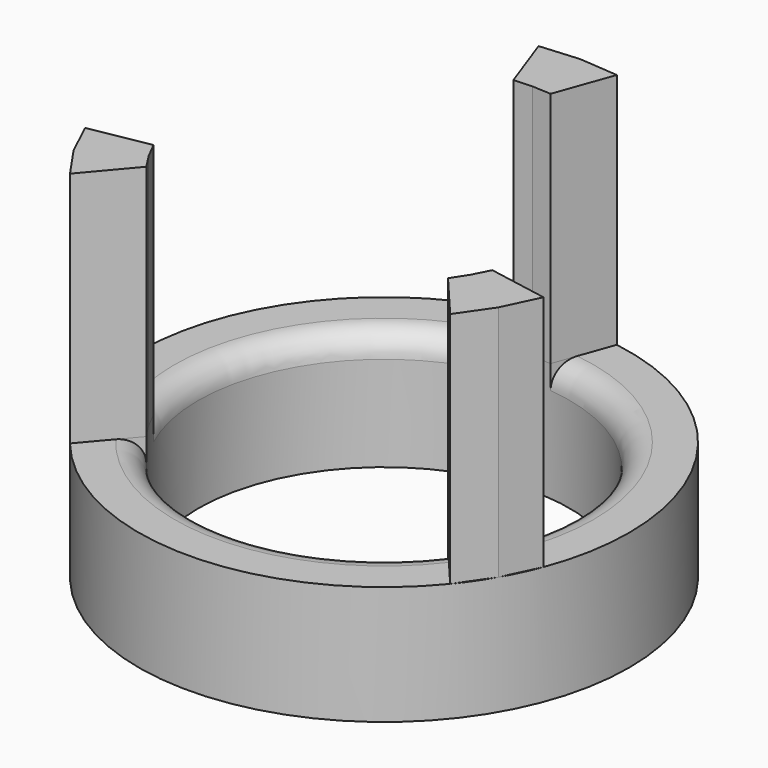
from build123d import *

# Parameters (mm, degrees)
F0_R         = 52.451
F0_R_2       = 39.751
F1_DEPTH     = 25.4
F3_DEPTH     = 50.8
F4_T4_ANGLE  = 145.1483416982
F4_T9_ANGLE  = 145.1483416982
F4_T16_ANGLE = 145.1483416982
F4_T23_ANGLE = 145.1483416982
F4_T28_ANGLE = 42.5640131775
F4_T33_ANGLE = 42.5640131775
F4_T38_ANGLE = 102.5699239424
F4_T44_ANGLE = 102.5699239424
F4_T49_ANGLE = 102.5699239424
F4_T54_ANGLE = 145.1483416982
F4_T59_ANGLE = 145.1483416982
F4_T66_ANGLE = 145.1483416982
F4_T73_ANGLE = 145.1483416982


# Not quite as in the source:
# - a fillet or chamfer that OpenCascade refuses, or shapes differently, is made with other operations: its cross-section is extruded or revolved along the edge and cut away or added


with BuildPart() as f1:
    # F0 (on Top) → F1 (new body)
    with BuildSketch(Plane.XY):
        Circle(F0_R)
        Circle(F0_R_2, mode=Mode.SUBTRACT)
    extrude(amount=F1_DEPTH)

    # F2 (on face) → F3 (join)
    with BuildSketch(Plane.XY.offset(25.4)):
        Polygon((0, 39.751), (3.9769716214, 39.5515574627), (8.3683463891, 51.7791288041), (0, 52.451), (-8.3683463891, 51.7791288041), (-3.9769716214, 39.5515574627), align=None)
        Polygon((-49.0262141247, -18.6423638414), (-45.4238984539, -26.2255), (-40.6578677356, -33.1367649627), (-32.2641677112, -23.2199371856), (-34.4253758258, -19.8755), (-36.2411393326, -16.331620277), align=None)
        Polygon((40.6578677356, -33.1367649627), (45.4238984539, -26.2255), (49.0262141247, -18.6423638414), (36.2411393326, -16.331620277), (34.4253758258, -19.8755), (32.2641677112, -23.2199371856), align=None)
    extrude(amount=F3_DEPTH)

    # F4: fillet of radius 5.08 on 4 edges, made by hand


with BuildPart() as f4_tool2:
    # F4_s3 → F4_t4 (revolve)
    with BuildSketch(Plane(origin=(0, 0, 0), x_dir=(0, 0, 1), z_dir=(0.9760150026, -0.2177032723, 0))):
        with BuildLine():
            ThreePointArc((25.4, -44.831), (23.9121024484, -41.2388975516), (20.32, -39.751))
            Line((20.32, -39.751), (25.4, -39.751))
            Line((25.4, -39.751), (25.4, -44.831))
        make_face()
    revolve(axis=Axis((0, 0, 25.4), (0, 0, 1)), revolution_arc=F4_T4_ANGLE)

    split(bisect_by=Plane(origin=(-9.0590317285, 3.2534345735, 0), x_dir=(0, 0, 1), z_dir=(0.9411459494, -0.3380004466, 0)), keep=Keep.TOP)


with BuildPart() as f1_1:
    add(f1.part)

    # F4_t1: cut F4_tool2
    add(f4_tool2.part, mode=Mode.SUBTRACT)


with BuildPart() as f4_tool7:
    # F4_s8 → F4_t9 (revolve)
    with BuildSketch(Plane(origin=(0, 0, 0), x_dir=(0, 0, 1), z_dir=(0.9760150026, -0.2177032723, 0))):
        with BuildLine():
            ThreePointArc((25.4, -44.831), (23.9121024484, -41.2388975516), (20.32, -39.751))
            Line((20.32, -39.751), (25.4, -39.751))
            Line((25.4, -39.751), (25.4, -44.831))
        make_face()
    revolve(axis=Axis((0, 0, 25.4), (0, 0, 1)), revolution_arc=F4_T9_ANGLE)

    split(bisect_by=Plane(origin=(9.0590317285, 3.2534345735, 0), x_dir=(0, 0, 1), z_dir=(-0.9411459494, -0.3380004466, 0)), keep=Keep.TOP)

    split(bisect_by=Plane(origin=(-33.3447717685, -21.5477185928, 0), x_dir=(0, 0, 1), z_dir=(0.8398952423, 0.542748544, 0)), keep=Keep.TOP)

    split(bisect_by=Plane(origin=(-35.3332575792, -18.1035601385, 0), x_dir=(0, 0, 1), z_dir=(0.8899816481, 0.4559963443, 0)), keep=Keep.TOP)


with BuildPart() as f1_2:
    add(f1_1.part)

    # F4_t6: cut F4_tool7
    add(f4_tool7.part, mode=Mode.SUBTRACT)


with BuildPart() as f4_tool14:
    # F4_s15 → F4_t16 (revolve)
    with BuildSketch(Plane(origin=(0, 0, 0), x_dir=(0, 0, 1), z_dir=(0.9760150026, -0.2177032723, 0))):
        with BuildLine():
            ThreePointArc((25.4, -44.831), (23.9121024484, -41.2388975516), (20.32, -39.751))
            Line((20.32, -39.751), (25.4, -39.751))
            Line((25.4, -39.751), (25.4, -44.831))
        make_face()
    revolve(axis=Axis((0, 0, 25.4), (0, 0, 1)), revolution_arc=F4_T16_ANGLE)

    split(bisect_by=Plane(origin=(1.7119588741, -9.4720688973, 0), x_dir=(0, 0, 1), z_dir=(-0.1778560014, 0.9840565242, 0)), keep=Keep.TOP)

    split(bisect_by=Plane(origin=(1.9884858107, 39.6512787313, 0), x_dir=(0, 0, 1), z_dir=(-0.0500864058, -0.9987448883, 0)), keep=Keep.TOP)

    split(bisect_by=Plane(origin=(-1.9884858107, 39.6512787313, 0), x_dir=(0, 0, 1), z_dir=(0.0500864058, -0.9987448883, 0)), keep=Keep.TOP)


with BuildPart() as f1_3:
    add(f1_2.part)

    # F4_t13: cut F4_tool14
    add(f4_tool14.part, mode=Mode.SUBTRACT)


with BuildPart() as f4_tool21:
    # F4_s22 → F4_t23 (revolve)
    with BuildSketch(Plane(origin=(0, 0, 0), x_dir=(0, 0, 1), z_dir=(0.9760150026, -0.2177032723, 0))):
        with BuildLine():
            ThreePointArc((25.4, -44.831), (23.9121024484, -41.2388975516), (20.32, -39.751))
            Line((20.32, -39.751), (25.4, -39.751))
            Line((25.4, -39.751), (25.4, -44.831))
        make_face()
    revolve(axis=Axis((0, 0, 25.4), (0, 0, 1)), revolution_arc=F4_T23_ANGLE)

    split(bisect_by=Plane(origin=(-7.3470728544, 6.2186343238, 0), x_dir=(0, 0, 1), z_dir=(0.763289948, -0.6460560775, 0)), keep=Keep.TOP)


with BuildPart() as f1_4:
    add(f1_3.part)

    # F4_t20: cut F4_tool21
    add(f4_tool21.part, mode=Mode.SUBTRACT)


with BuildPart() as f4_tool26:
    # F4_s27 → F4_t28 (revolve)
    with BuildSketch(Plane(origin=(0, 0, 0), x_dir=(0, 0, 1), z_dir=(-0.6764135021, -0.7365220799, 0))):
        with BuildLine():
            ThreePointArc((25.4, -44.831), (23.9121024484, -41.2388975516), (20.32, -39.751))
            Line((20.32, -39.751), (25.4, -39.751))
            Line((25.4, -39.751), (25.4, -44.831))
        make_face()
    revolve(axis=Axis((0, 0, 25.4), (0, 0, 1)), revolution_arc=F4_T28_ANGLE)

    split(bisect_by=Plane(origin=(7.3470728544, 6.2186343238, 0), x_dir=(0, 0, 1), z_dir=(-0.763289948, -0.6460560775, 0)), keep=Keep.TOP)


with BuildPart() as f1_5:
    add(f1_4.part)

    # F4_t25: cut F4_tool26
    add(f4_tool26.part, mode=Mode.SUBTRACT)


with BuildPart() as f4_tool31:
    # F4_s32 → F4_t33 (revolve)
    with BuildSketch(Plane(origin=(0, 0, 0), x_dir=(0, 0, 1), z_dir=(-0.6764135021, -0.7365220799, 0))):
        with BuildLine():
            ThreePointArc((25.4, -44.831), (23.9121024484, -41.2388975516), (20.32, -39.751))
            Line((20.32, -39.751), (25.4, -39.751))
            Line((25.4, -39.751), (25.4, -44.831))
        make_face()
    revolve(axis=Axis((0, 0, 25.4), (0, 0, 1)), revolution_arc=F4_T33_ANGLE)

    split(bisect_by=Plane(origin=(-1.7119588741, -9.4720688973, 0), x_dir=(0, 0, 1), z_dir=(0.1778560014, 0.9840565242, 0)), keep=Keep.TOP)


with BuildPart() as f1_6:
    add(f1_5.part)

    # F4_t30: cut F4_tool31
    add(f4_tool31.part, mode=Mode.SUBTRACT)


with BuildPart() as f4_tool36:
    # F4_s37 → F4_t38 (revolve)
    with BuildSketch(Plane.XZ):
        with BuildLine():
            ThreePointArc((44.831, 25.4), (41.2388975516, 23.9121024484), (39.751, 20.32))
            Line((39.751, 20.32), (39.751, 25.4))
            Line((39.751, 25.4), (44.831, 25.4))
        make_face()
    revolve(axis=Axis((0, 0, 25.4), (0, 0, 1)), revolution_arc=F4_T38_ANGLE)

    split(bisect_by=Plane(origin=(1.9884858107, 39.6512787313, 0), x_dir=(0, 0, 1), z_dir=(-0.0500864058, -0.9987448883, 0)), keep=Keep.TOP)

    split(bisect_by=Plane(origin=(-1.9884858107, 39.6512787313, 0), x_dir=(0, 0, 1), z_dir=(0.0500864058, -0.9987448883, 0)), keep=Keep.TOP)


with BuildPart() as f1_7:
    add(f1_6.part)

    # F4_t35: cut F4_tool36
    add(f4_tool36.part, mode=Mode.SUBTRACT)


with BuildPart() as f4_tool42:
    # F4_s43 → F4_t44 (revolve)
    with BuildSketch(Plane.XZ):
        with BuildLine():
            ThreePointArc((44.831, 25.4), (41.2388975516, 23.9121024484), (39.751, 20.32))
            Line((39.751, 20.32), (39.751, 25.4))
            Line((39.751, 25.4), (44.831, 25.4))
        make_face()
    revolve(axis=Axis((0, 0, 25.4), (0, 0, 1)), revolution_arc=F4_T44_ANGLE)

    split(bisect_by=Plane(origin=(-9.0590317285, 3.2534345735, 0), x_dir=(0, 0, 1), z_dir=(0.9411459494, -0.3380004466, 0)), keep=Keep.TOP)


with BuildPart() as f1_8:
    add(f1_7.part)

    # F4_t41: cut F4_tool42
    add(f4_tool42.part, mode=Mode.SUBTRACT)


with BuildPart() as f4_tool47:
    # F4_s48 → F4_t49 (revolve)
    with BuildSketch(Plane.XZ):
        with BuildLine():
            ThreePointArc((44.831, 25.4), (41.2388975516, 23.9121024484), (39.751, 20.32))
            Line((39.751, 20.32), (39.751, 25.4))
            Line((39.751, 25.4), (44.831, 25.4))
        make_face()
    revolve(axis=Axis((0, 0, 25.4), (0, 0, 1)), revolution_arc=F4_T49_ANGLE)

    split(bisect_by=Plane(origin=(9.0590317285, 3.2534345735, 0), x_dir=(0, 0, 1), z_dir=(-0.9411459494, -0.3380004466, 0)), keep=Keep.TOP)


with BuildPart() as f1_9:
    add(f1_8.part)

    # F4_t46: cut F4_tool47
    add(f4_tool47.part, mode=Mode.SUBTRACT)


with BuildPart() as f4_tool52:
    # F4_s53 → F4_t54 (revolve)
    with BuildSketch(Plane(origin=(0, 0, 0), x_dir=(0, 0, 1), z_dir=(-0.299470937, 0.9541054229, 0))):
        with BuildLine():
            ThreePointArc((25.4, -44.831), (23.9121024484, -41.2388975516), (20.32, -39.751))
            Line((20.32, -39.751), (25.4, -39.751))
            Line((25.4, -39.751), (25.4, -44.831))
        make_face()
    revolve(axis=Axis((0, 0, 25.4), (0, 0, 1)), revolution_arc=F4_T54_ANGLE)

    split(bisect_by=Plane(origin=(1.7119588741, -9.4720688973, 0), x_dir=(0, 0, 1), z_dir=(-0.1778560014, 0.9840565242, 0)), keep=Keep.TOP)


with BuildPart() as f1_10:
    add(f1_9.part)

    # F4_t51: cut F4_tool52
    add(f4_tool52.part, mode=Mode.SUBTRACT)


with BuildPart() as f4_tool57:
    # F4_s58 → F4_t59 (revolve)
    with BuildSketch(Plane(origin=(0, 0, 0), x_dir=(0, 0, 1), z_dir=(-0.299470937, 0.9541054229, 0))):
        with BuildLine():
            ThreePointArc((25.4, -44.831), (23.9121024484, -41.2388975516), (20.32, -39.751))
            Line((20.32, -39.751), (25.4, -39.751))
            Line((25.4, -39.751), (25.4, -44.831))
        make_face()
    revolve(axis=Axis((0, 0, 25.4), (0, 0, 1)), revolution_arc=F4_T59_ANGLE)

    split(bisect_by=Plane(origin=(-7.3470728544, 6.2186343238, 0), x_dir=(0, 0, 1), z_dir=(0.763289948, -0.6460560775, 0)), keep=Keep.TOP)

    split(bisect_by=Plane(origin=(35.3332575792, -18.1035601385, 0), x_dir=(0, 0, 1), z_dir=(-0.8899816481, 0.4559963443, 0)), keep=Keep.TOP)

    split(bisect_by=Plane(origin=(33.3447717685, -21.5477185928, 0), x_dir=(0, 0, 1), z_dir=(-0.8398952423, 0.542748544, 0)), keep=Keep.TOP)


with BuildPart() as f1_11:
    add(f1_10.part)

    # F4_t56: cut F4_tool57
    add(f4_tool57.part, mode=Mode.SUBTRACT)


with BuildPart() as f4_tool64:
    # F4_s65 → F4_t66 (revolve)
    with BuildSketch(Plane(origin=(0, 0, 0), x_dir=(0, 0, 1), z_dir=(-0.299470937, 0.9541054229, 0))):
        with BuildLine():
            ThreePointArc((25.4, -44.831), (23.9121024484, -41.2388975516), (20.32, -39.751))
            Line((20.32, -39.751), (25.4, -39.751))
            Line((25.4, -39.751), (25.4, -44.831))
        make_face()
    revolve(axis=Axis((0, 0, 25.4), (0, 0, 1)), revolution_arc=F4_T66_ANGLE)

    split(bisect_by=Plane(origin=(7.3470728544, 6.2186343238, 0), x_dir=(0, 0, 1), z_dir=(-0.763289948, -0.6460560775, 0)), keep=Keep.TOP)

    split(bisect_by=Plane(origin=(-33.3447717685, -21.5477185928, 0), x_dir=(0, 0, 1), z_dir=(0.8398952423, 0.542748544, 0)), keep=Keep.TOP)

    split(bisect_by=Plane(origin=(-35.3332575792, -18.1035601385, 0), x_dir=(0, 0, 1), z_dir=(0.8899816481, 0.4559963443, 0)), keep=Keep.TOP)


with BuildPart() as f1_12:
    add(f1_11.part)

    # F4_t63: cut F4_tool64
    add(f4_tool64.part, mode=Mode.SUBTRACT)


with BuildPart() as f4_tool71:
    # F4_s72 → F4_t73 (revolve)
    with BuildSketch(Plane(origin=(0, 0, 0), x_dir=(0, 0, 1), z_dir=(-0.299470937, 0.9541054229, 0))):
        with BuildLine():
            ThreePointArc((25.4, -44.831), (23.9121024484, -41.2388975516), (20.32, -39.751))
            Line((20.32, -39.751), (25.4, -39.751))
            Line((25.4, -39.751), (25.4, -44.831))
        make_face()
    revolve(axis=Axis((0, 0, 25.4), (0, 0, 1)), revolution_arc=F4_T73_ANGLE)

    split(bisect_by=Plane(origin=(-1.7119588741, -9.4720688973, 0), x_dir=(0, 0, 1), z_dir=(0.1778560014, 0.9840565242, 0)), keep=Keep.TOP)


with BuildPart() as f1_13:
    add(f1_12.part)

    # F4_t70: cut F4_tool71
    add(f4_tool71.part, mode=Mode.SUBTRACT)


solid = f1_13.part
